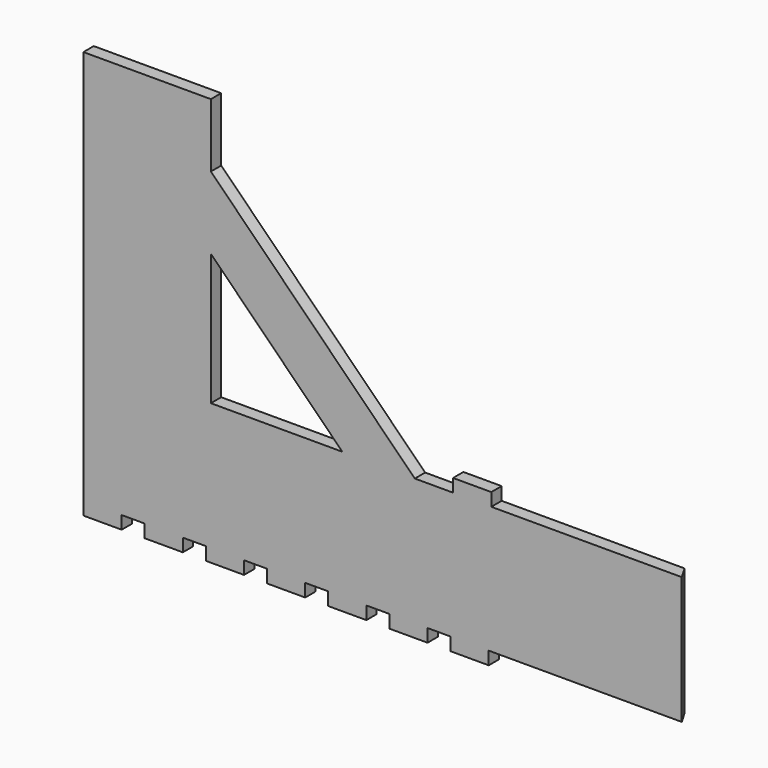
from build123d import *

# Parameters (mm, degrees)
F0_W     = 15
F0_H     = 5.08
F1_DEPTH = 5.08
F2_DEPTH = 25
F4_DEPTH = 50
F5_W     = 15
F5_H     = 5.08
F6_DEPTH = 5.08


# Not quite as in the source:
# - a feature names something its author has since deleted; it is built from what else it names


with BuildPart() as f1:
    # F0 (on Front) → F1 (new body)
    with BuildSketch(Plane.XZ):
        Polygon((-75.7, 0), (0, 0), (0, 50), (-104.7, 50), (-133.1023774395, 50), (-184.7, 50), (-184.7, 101.5976225605), (-184.7, 130), (-234.7, 130), (-234.7, 0), (-219.7, 0), (-210.7, 0), (-195.7, 0), (-186.7, 0), (-171.7, 0), (-162.7, 0), (-147.7, 0), (-138.7, 0), (-123.7, 0), (-114.7, 0), (-99.7, 0), (-90.7, 0), align=None)
        with Locations((-83.2, -2.54)):
            Rectangle(F0_W, F0_H)
        Polygon((-133.1023774395, 50), (-104.7, 50), (-184.7, 130), (-184.7, 101.5976225605), align=None)
        with Locations((-107.2, -2.54)):
            Rectangle(F0_W, F0_H)
        with Locations((-131.2, -2.54)):
            Rectangle(F0_W, F0_H)
        with Locations((-227.2, -2.54)):
            Rectangle(F0_W, F0_H)
        with Locations((-155.2, -2.54)):
            Rectangle(F0_W, F0_H)
        with Locations((-203.2, -2.54)):
            Rectangle(F0_W, F0_H)
        with Locations((-179.2, -2.54)):
            Rectangle(F0_W, F0_H)
    extrude(amount=F1_DEPTH)

    # F2 (add): a face of the model
    f2_faces = [f1.faces().sort_by_distance(p)[0] for p in [
        (-209.7, -2.54, 130),
    ]]
    extrude(f2_faces, amount=F2_DEPTH)

    # F3 (on face) → F4 (cut)
    with BuildSketch(Plane(origin=(0, 0, 0), x_dir=(1, 0, 0), z_dir=(0, 0, -1))):
        Polygon((0, 0), (0, 5.08), (-2.9329393675, 0), align=None)
    extrude(amount=-F4_DEPTH, mode=Mode.SUBTRACT)

    # F5 (on face) → F6 (join)
    with BuildSketch(Plane.XY.offset(50)):
        with Locations((-82.2, -2.54)):
            Rectangle(F5_W, F5_H)
    extrude(amount=F6_DEPTH)


solid = f1.part
